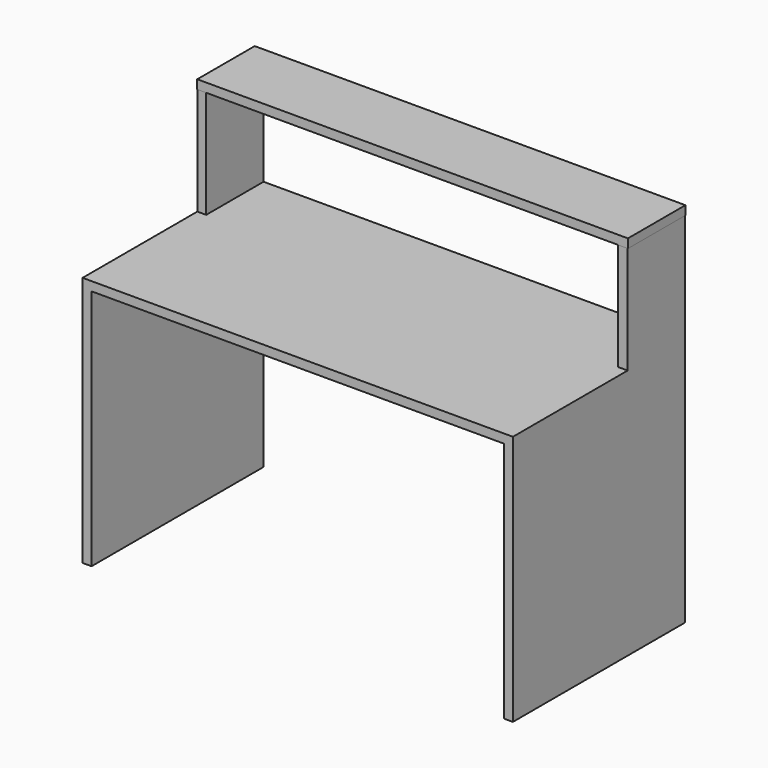
from build123d import *

# Parameters (mm, degrees)
F0_W     = 1200
F0_H     = 600
F1_DEPTH = 25
F2_W     = 25
F2_H     = 600
F3_DEPTH = 675
F4_W     = 24.7376918793
F4_H     = 200
F4_W_2   = 26.8032312393
F5_DEPTH = 300
F6_W     = 24.7376918793
F6_H     = 200
F7_DEPTH = 25


with BuildPart() as f1:
    # F0 (on Top) → F1 (new body)
    with BuildSketch(Plane.XY):
        Rectangle(F0_W, F0_H)
    extrude(amount=F1_DEPTH)

    # F2 (on face) → F3 (join)
    with BuildSketch(Plane(origin=(0, 0, 0), x_dir=(1, 0, 0), z_dir=(0, 0, -1))):
        with Locations((-587.5, 0)):
            Rectangle(F2_W, F2_H)
        with Locations((587.5, 0)):
            Rectangle(F2_W, F2_H)
    extrude(amount=F3_DEPTH)

    # F4 (on face) → F5 (join)
    with BuildSketch(Plane.XY.offset(25)):
        with Locations((-587.6311540604, 200)):
            Rectangle(F4_W, F4_H)
        with Locations((586.5983843803, 200)):
            Rectangle(F4_W_2, F4_H)
    extrude(amount=F5_DEPTH)

    # F6 (on face) → F7 (join)
    with BuildSketch(Plane.XY.offset(325)):
        with Locations((-587.6311540604, 200)):
            Rectangle(F6_W, F6_H)
        Polygon((601.0820269585, 300), (-575.2623081207, 300), (-575.2623081207, 100), (-600, 100), (-600, 99.6639356017), (601.0820269585, 99.6639356017), align=None)
    extrude(amount=F7_DEPTH)


solid = f1.part
